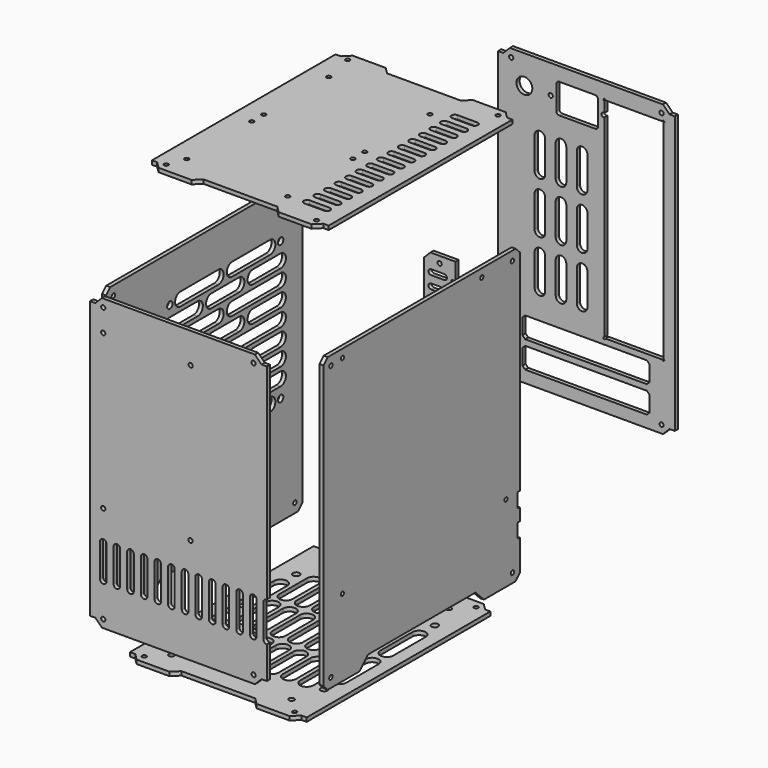
from build123d import *

# Parameters (mm, degrees)
F0_R      = 1.6
F1_DEPTH  = 3
F3_R      = 1.6
F4_DEPTH  = 3
F6_R      = 1.6
F7_DEPTH  = 3
F9_R      = 1.5
F9_W      = 2
F9_H      = 11
F10_DEPTH = 25
F12_R     = 1.6
F13_DEPTH = 3
F15_R     = 2.55
F16_DEPTH = 25
F18_R     = 1.6
F19_DEPTH = 3
F22_R     = 1.6
F23_DEPTH = 3
F26_R     = 1.6
F27_DEPTH = 3
F29_W     = 96.4
F29_H     = 15.9
F30_R     = 6
F30_R_2   = 1.6
F31_DEPTH = 25
F32_SIZE  = 2
F33_R     = 1.6
F34_DEPTH = 25
F35_R     = 2.55
F35_R_2   = 2
F36_DEPTH = 25
F37_R     = 1.6
F38_DEPTH = 3
F39_SIZE  = 0.5


# Not quite as in the source:
# - a feature names something its author has since deleted; it is built from what else it names


with BuildPart() as f1:
    # F0 (on Front) → F1 (new body)
    with BuildSketch(Plane.XZ):
        Polygon((-72.4445467208, 96.6760702261), (-76.4445467208, 96.6760702261), (-76.4445467208, -8.3239297739), (57.5554532792, -8.3239297739), (57.5554532792, 96.6760702261), (53.5554532792, 96.6760702261), (48.5554532792, 101.6760702261), (-67.4445467208, 101.6760702261), align=None)
        with Locations((-66.4445467208, 95.6760702261)):
            Circle(F0_R, mode=Mode.SUBTRACT)
        with Locations((47.5554532792, 95.6760702261)):
            Circle(F0_R, mode=Mode.SUBTRACT)
    extrude(amount=F1_DEPTH)

    # F2: F1 across face


with BuildPart() as f1_1:
    add(f1.part)
    add(f1.part.mirror(Plane(origin=(-9.4445467208, -1.5, -8.3239297739), x_dir=(1, 0, 0), z_dir=(0, 0, -1))))

    # F3 (on face) → F4 (cut)
    with BuildSketch(Plane.XZ.offset(3)):
        with Locations((-0.2445467208, 78.6760702261)):
            Circle(F3_R)
        with Locations((-66.4445467208, 78.6760702261)):
            Circle(F3_R)
        with Locations((-66.4445467208, -38.3239297739)):
            Circle(F3_R)
        with Locations((-0.2445467208, -38.3239297739)):
            Circle(F3_R)
        with BuildLine():
            ThreePointArc((-68.9445467208, -86.3239297739), (-66.4445467208, -88.8239297739), (-63.9445467208, -86.3239297739))
            Line((-63.9445467208, -86.3239297739), (-63.9445467208, -61.3239297739))
            ThreePointArc((-63.9445467208, -61.3239297739), (-66.4445467208, -58.8239297739), (-68.9445467208, -61.3239297739))
            Line((-68.9445467208, -61.3239297739), (-68.9445467208, -86.3239297739))
        make_face()
        with BuildLine():
            ThreePointArc((-58.6115467208, -86.3239297739), (-56.1115467208, -88.8239297739), (-53.6115467208, -86.3239297739))
            Line((-53.6115467208, -86.3239297739), (-53.6115467208, -61.3239297739))
            ThreePointArc((-53.6115467208, -61.3239297739), (-56.1115467208, -58.8239297739), (-58.6115467208, -61.3239297739))
            Line((-58.6115467208, -61.3239297739), (-58.6115467208, -86.3239297739))
        make_face()
        with BuildLine():
            ThreePointArc((-48.2785467208, -86.3239297739), (-45.7785467208, -88.8239297739), (-43.2785467208, -86.3239297739))
            Line((-43.2785467208, -86.3239297739), (-43.2785467208, -61.3239297739))
            ThreePointArc((-43.2785467208, -61.3239297739), (-45.7785467208, -58.8239297739), (-48.2785467208, -61.3239297739))
            Line((-48.2785467208, -61.3239297739), (-48.2785467208, -86.3239297739))
        make_face()
        with BuildLine():
            ThreePointArc((-37.9455467208, -86.3239297739), (-35.4455467208, -88.8239297739), (-32.9455467208, -86.3239297739))
            Line((-32.9455467208, -86.3239297739), (-32.9455467208, -61.3239297739))
            ThreePointArc((-32.9455467208, -61.3239297739), (-35.4455467208, -58.8239297739), (-37.9455467208, -61.3239297739))
            Line((-37.9455467208, -61.3239297739), (-37.9455467208, -86.3239297739))
        make_face()
        with BuildLine():
            ThreePointArc((-27.6125467208, -86.3239297739), (-25.1125467208, -88.8239297739), (-22.6125467208, -86.3239297739))
            Line((-22.6125467208, -86.3239297739), (-22.6125467208, -61.3239297739))
            ThreePointArc((-22.6125467208, -61.3239297739), (-25.1125467208, -58.8239297739), (-27.6125467208, -61.3239297739))
            Line((-27.6125467208, -61.3239297739), (-27.6125467208, -86.3239297739))
        make_face()
        with BuildLine():
            ThreePointArc((-17.2795467208, -86.3239297739), (-14.7795467208, -88.8239297739), (-12.2795467208, -86.3239297739))
            Line((-12.2795467208, -86.3239297739), (-12.2795467208, -61.3239297739))
            ThreePointArc((-12.2795467208, -61.3239297739), (-14.7795467208, -58.8239297739), (-17.2795467208, -61.3239297739))
            Line((-17.2795467208, -61.3239297739), (-17.2795467208, -86.3239297739))
        make_face()
        with BuildLine():
            ThreePointArc((-6.9465467208, -86.3239297739), (-4.4465467208, -88.8239297739), (-1.9465467208, -86.3239297739))
            Line((-1.9465467208, -86.3239297739), (-1.9465467208, -61.3239297739))
            ThreePointArc((-1.9465467208, -61.3239297739), (-4.4465467208, -58.8239297739), (-6.9465467208, -61.3239297739))
            Line((-6.9465467208, -61.3239297739), (-6.9465467208, -86.3239297739))
        make_face()
        with BuildLine():
            ThreePointArc((3.3864532792, -86.3239297739), (5.8864532792, -88.8239297739), (8.3864532792, -86.3239297739))
            Line((8.3864532792, -86.3239297739), (8.3864532792, -61.3239297739))
            ThreePointArc((8.3864532792, -61.3239297739), (5.8864532792, -58.8239297739), (3.3864532792, -61.3239297739))
            Line((3.3864532792, -61.3239297739), (3.3864532792, -86.3239297739))
        make_face()
        with BuildLine():
            ThreePointArc((13.7194532792, -86.3239297739), (16.2194532792, -88.8239297739), (18.7194532792, -86.3239297739))
            Line((18.7194532792, -86.3239297739), (18.7194532792, -61.3239297739))
            ThreePointArc((18.7194532792, -61.3239297739), (16.2194532792, -58.8239297739), (13.7194532792, -61.3239297739))
            Line((13.7194532792, -61.3239297739), (13.7194532792, -86.3239297739))
        make_face()
        with BuildLine():
            ThreePointArc((24.0524532792, -86.3239297739), (26.5524532792, -88.8239297739), (29.0524532792, -86.3239297739))
            Line((29.0524532792, -86.3239297739), (29.0524532792, -61.3239297739))
            ThreePointArc((29.0524532792, -61.3239297739), (26.5524532792, -58.8239297739), (24.0524532792, -61.3239297739))
            Line((24.0524532792, -61.3239297739), (24.0524532792, -86.3239297739))
        make_face()
        with BuildLine():
            ThreePointArc((34.3854532792, -86.3239297739), (36.8854532792, -88.8239297739), (39.3854532792, -86.3239297739))
            Line((39.3854532792, -86.3239297739), (39.3854532792, -61.3239297739))
            ThreePointArc((39.3854532792, -61.3239297739), (36.8854532792, -58.8239297739), (34.3854532792, -61.3239297739))
            Line((34.3854532792, -61.3239297739), (34.3854532792, -86.3239297739))
        make_face()
        with BuildLine():
            ThreePointArc((44.7184532792, -86.3239297739), (47.2184532792, -88.8239297739), (49.7184532792, -86.3239297739))
            Line((49.7184532792, -86.3239297739), (49.7184532792, -61.3239297739))
            ThreePointArc((49.7184532792, -61.3239297739), (47.2184532792, -58.8239297739), (44.7184532792, -61.3239297739))
            Line((44.7184532792, -61.3239297739), (44.7184532792, -86.3239297739))
        make_face()
        with BuildLine():
            ThreePointArc((55.0514532792, -86.3239297739), (57.5514532792, -88.8239297739), (60.0514532792, -86.3239297739))
            Line((60.0514532792, -86.3239297739), (60.0514532792, -61.3239297739))
            ThreePointArc((60.0514532792, -61.3239297739), (57.5514532792, -58.8239297739), (55.0514532792, -61.3239297739))
            Line((55.0514532792, -61.3239297739), (55.0514532792, -86.3239297739))
        make_face()
    extrude(amount=-F4_DEPTH, mode=Mode.SUBTRACT)


with BuildPart() as f7:
    # F6 (on offset) → F7 (new body)
    with BuildSketch(Plane.YZ.offset(80)):
        Polygon((200.9140200328, 100.6278687119), (22.9140200328, 100.6278687119), (18.9140200328, 96.6278687119), (18.9140200328, -10.3721312881), (204.9140200328, -10.3721312881), (204.9140200328, 96.6278687119), align=None)
        with Locations((25.9140200328, 93.6278687119)):
            Circle(F6_R, mode=Mode.SUBTRACT)
        with Locations((197.9140200328, 93.6278687119)):
            Circle(F6_R, mode=Mode.SUBTRACT)
    extrude(amount=F7_DEPTH)

    # F8: F7 across face


with BuildPart() as f7_1:
    add(f7.part)
    add(f7.part.mirror(Plane(origin=(81.5, 111.9140200328, -10.3721312881), x_dir=(1, 0, 0), z_dir=(0, 0, -1))))

    # F9 (on face) → F10 (cut)
    with BuildSketch(Plane(origin=(80, 0, 0), x_dir=(0, -1, 0), z_dir=(-1, 0, 0))):
        with Locations((-191.7140200328, -62.9721312881)):
            Circle(F9_R)
        with Locations((-36.8140200328, -62.9721312881)):
            Circle(F9_R)
        with Locations((-168.9140200328, 94.4278687119)):
            Circle(F9_R)
        with Locations((-36.8140200328, 94.4278687119)):
            Circle(F9_R)
        Polygon((-170.9140200328, -121.3721312881), (-52.9140200328, -121.3721312881), (-60.9140200328, -113.3721312881), (-162.9140200328, -113.3721312881), align=None)
        with Locations((-203.9140200328, -68.0721312881)):
            Rectangle(F9_W, F9_H)
        with Locations((-203.9140200328, -88.3721312881)):
            Rectangle(F9_W, F9_H)
    extrude(amount=-F10_DEPTH, mode=Mode.SUBTRACT)

    # F39
    f39_edges = [f7_1.edges().sort_by_distance(p)[0] for p in [
        (81.5, 202.91402, -93.872131),
        (81.5, 202.91402, -73.572131),
        (81.5, 202.91402, -62.572131),
        (81.5, 202.91402, -82.872131),
    ]]
    chamfer(f39_edges, length=F39_SIZE)


with BuildPart() as f13:
    # F12 (on offset) → F13 (new body)
    with BuildSketch(Plane.YZ.offset(-96)):
        Polygon((218.7864820957, 80.4807467597), (214.7864820957, 84.4807467597), (36.7864820957, 84.4807467597), (32.7864820957, 80.4807467597), (32.7864820957, -26.5192532403), (218.7864820957, -26.5192532403), align=None)
        with Locations((39.7864820957, 77.4807467597)):
            Circle(F12_R, mode=Mode.SUBTRACT)
        with Locations((211.7864820957, 77.4807467597)):
            Circle(F12_R, mode=Mode.SUBTRACT)
    extrude(amount=F13_DEPTH)

    # F14: F13 across face


with BuildPart() as f13_1:
    add(f13.part)
    add(f13.part.mirror(Plane(origin=(-94.5, 125.7864820957, -26.5192532403), x_dir=(1, 0, 0), z_dir=(0, 0, -1))))

    # F15 (on face) → F16 (cut)
    with BuildSketch(Plane(origin=(-96, 0, 0), x_dir=(0, -1, 0), z_dir=(-1, 0, 0))):
        with Locations((-198.2864820957, 49.4807467597)):
            Circle(F15_R)
        with Locations((-93.2864820957, 49.4807467597)):
            Circle(F15_R)
        with BuildLine():
            ThreePointArc((-188.2864820957, 54.4807467597), (-193.2864820957, 49.4807467597), (-188.2864820957, 44.4807467597))
            Line((-188.2864820957, 44.4807467597), (-152.2864820957, 44.4807467597))
            ThreePointArc((-152.2864820957, 44.4807467597), (-147.2864820957, 49.4807467597), (-152.2864820957, 54.4807467597))
            Line((-152.2864820957, 54.4807467597), (-188.2864820957, 54.4807467597))
        make_face()
        with BuildLine():
            ThreePointArc((-139.2864820957, 54.4807467597), (-144.2864820957, 49.4807467597), (-139.2864820957, 44.4807467597))
            Line((-139.2864820957, 44.4807467597), (-103.2864820957, 44.4807467597))
            ThreePointArc((-103.2864820957, 44.4807467597), (-98.2864820957, 49.4807467597), (-103.2864820957, 54.4807467597))
            Line((-103.2864820957, 54.4807467597), (-139.2864820957, 54.4807467597))
        make_face()
        with BuildLine():
            ThreePointArc((-198.2864820957, 41.3557467597), (-203.2864820957, 36.3557467597), (-198.2864820957, 31.3557467597))
            Line((-198.2864820957, 31.3557467597), (-171.9531487624, 31.3557467597))
            ThreePointArc((-171.9531487624, 31.3557467597), (-166.9531487624, 36.3557467597), (-171.9531487624, 41.3557467597))
            Line((-171.9531487624, 41.3557467597), (-198.2864820957, 41.3557467597))
        make_face()
        with BuildLine():
            ThreePointArc((-158.9531487624, 41.3557467597), (-163.9531487624, 36.3557467597), (-158.9531487624, 31.3557467597))
            Line((-158.9531487624, 31.3557467597), (-132.6198154291, 31.3557467597))
            ThreePointArc((-132.6198154291, 31.3557467597), (-127.6198154291, 36.3557467597), (-132.6198154291, 41.3557467597))
            Line((-132.6198154291, 41.3557467597), (-158.9531487624, 41.3557467597))
        make_face()
        with BuildLine():
            ThreePointArc((-119.6198154291, 41.3557467597), (-124.6198154291, 36.3557467597), (-119.6198154291, 31.3557467597))
            Line((-119.6198154291, 31.3557467597), (-93.2864820957, 31.3557467597))
            ThreePointArc((-93.2864820957, 31.3557467597), (-88.2864820957, 36.3557467597), (-93.2864820957, 41.3557467597))
            Line((-93.2864820957, 41.3557467597), (-119.6198154291, 41.3557467597))
        make_face()
        with BuildLine():
            ThreePointArc((-198.2864820957, 28.2307467597), (-203.2864820957, 23.2307467597), (-198.2864820957, 18.2307467597))
            Line((-198.2864820957, 18.2307467597), (-152.2864820957, 18.2307467597))
            ThreePointArc((-152.2864820957, 18.2307467597), (-147.2864820957, 23.2307467597), (-152.2864820957, 28.2307467597))
            Line((-152.2864820957, 28.2307467597), (-198.2864820957, 28.2307467597))
        make_face()
        with BuildLine():
            ThreePointArc((-139.2864820957, 28.2307467597), (-144.2864820957, 23.2307467597), (-139.2864820957, 18.2307467597))
            Line((-139.2864820957, 18.2307467597), (-93.2864820957, 18.2307467597))
            ThreePointArc((-93.2864820957, 18.2307467597), (-88.2864820957, 23.2307467597), (-93.2864820957, 28.2307467597))
            Line((-93.2864820957, 28.2307467597), (-139.2864820957, 28.2307467597))
        make_face()
        with BuildLine():
            ThreePointArc((-198.2864820957, 15.1057467597), (-203.2864820957, 10.1057467597), (-198.2864820957, 5.1057467597))
            Line((-198.2864820957, 5.1057467597), (-171.9531487624, 5.1057467597))
            ThreePointArc((-171.9531487624, 5.1057467597), (-166.9531487624, 10.1057467597), (-171.9531487624, 15.1057467597))
            Line((-171.9531487624, 15.1057467597), (-198.2864820957, 15.1057467597))
        make_face()
        with BuildLine():
            ThreePointArc((-158.9531487624, 15.1057467597), (-163.9531487624, 10.1057467597), (-158.9531487624, 5.1057467597))
            Line((-158.9531487624, 5.1057467597), (-132.6198154291, 5.1057467597))
            ThreePointArc((-132.6198154291, 5.1057467597), (-127.6198154291, 10.1057467597), (-132.6198154291, 15.1057467597))
            Line((-132.6198154291, 15.1057467597), (-158.9531487624, 15.1057467597))
        make_face()
        with BuildLine():
            ThreePointArc((-119.6198154291, 15.1057467597), (-124.6198154291, 10.1057467597), (-119.6198154291, 5.1057467597))
            Line((-119.6198154291, 5.1057467597), (-93.2864820957, 5.1057467597))
            ThreePointArc((-93.2864820957, 5.1057467597), (-88.2864820957, 10.1057467597), (-93.2864820957, 15.1057467597))
            Line((-93.2864820957, 15.1057467597), (-119.6198154291, 15.1057467597))
        make_face()
        with BuildLine():
            ThreePointArc((-198.2864820957, 1.9807467597), (-203.2864820957, -3.0192532403), (-198.2864820957, -8.0192532403))
            Line((-198.2864820957, -8.0192532403), (-152.2864820957, -8.0192532403))
            ThreePointArc((-152.2864820957, -8.0192532403), (-147.2864820957, -3.0192532403), (-152.2864820957, 1.9807467597))
            Line((-152.2864820957, 1.9807467597), (-198.2864820957, 1.9807467597))
        make_face()
        with BuildLine():
            ThreePointArc((-139.2864820957, 1.9807467597), (-144.2864820957, -3.0192532403), (-139.2864820957, -8.0192532403))
            Line((-139.2864820957, -8.0192532403), (-93.2864820957, -8.0192532403))
            ThreePointArc((-93.2864820957, -8.0192532403), (-88.2864820957, -3.0192532403), (-93.2864820957, 1.9807467597))
            Line((-93.2864820957, 1.9807467597), (-139.2864820957, 1.9807467597))
        make_face()
        with BuildLine():
            ThreePointArc((-198.2864820957, -11.1442532403), (-203.2864820957, -16.1442532403), (-198.2864820957, -21.1442532403))
            Line((-198.2864820957, -21.1442532403), (-171.9531487624, -21.1442532403))
            ThreePointArc((-171.9531487624, -21.1442532403), (-166.9531487624, -16.1442532403), (-171.9531487624, -11.1442532403))
            Line((-171.9531487624, -11.1442532403), (-198.2864820957, -11.1442532403))
        make_face()
        with BuildLine():
            ThreePointArc((-158.9531487624, -11.1442532403), (-163.9531487624, -16.1442532403), (-158.9531487624, -21.1442532403))
            Line((-158.9531487624, -21.1442532403), (-132.6198154291, -21.1442532403))
            ThreePointArc((-132.6198154291, -21.1442532403), (-127.6198154291, -16.1442532403), (-132.6198154291, -11.1442532403))
            Line((-132.6198154291, -11.1442532403), (-158.9531487624, -11.1442532403))
        make_face()
        with BuildLine():
            ThreePointArc((-119.6198154291, -11.1442532403), (-124.6198154291, -16.1442532403), (-119.6198154291, -21.1442532403))
            Line((-119.6198154291, -21.1442532403), (-93.2864820957, -21.1442532403))
            ThreePointArc((-93.2864820957, -21.1442532403), (-88.2864820957, -16.1442532403), (-93.2864820957, -11.1442532403))
            Line((-93.2864820957, -11.1442532403), (-119.6198154291, -11.1442532403))
        make_face()
        with BuildLine():
            ThreePointArc((-198.2864820957, -24.2692532403), (-203.2864820957, -29.2692532403), (-198.2864820957, -34.2692532403))
            Line((-198.2864820957, -34.2692532403), (-152.2864820957, -34.2692532403))
            ThreePointArc((-152.2864820957, -34.2692532403), (-147.2864820957, -29.2692532403), (-152.2864820957, -24.2692532403))
            Line((-152.2864820957, -24.2692532403), (-198.2864820957, -24.2692532403))
        make_face()
        with BuildLine():
            ThreePointArc((-139.2864820957, -24.2692532403), (-144.2864820957, -29.2692532403), (-139.2864820957, -34.2692532403))
            Line((-139.2864820957, -34.2692532403), (-93.2864820957, -34.2692532403))
            ThreePointArc((-93.2864820957, -34.2692532403), (-88.2864820957, -29.2692532403), (-93.2864820957, -24.2692532403))
            Line((-93.2864820957, -24.2692532403), (-139.2864820957, -24.2692532403))
        make_face()
        with BuildLine():
            ThreePointArc((-198.2864820957, -37.3942532403), (-203.2864820957, -42.3942532403), (-198.2864820957, -47.3942532403))
            Line((-198.2864820957, -47.3942532403), (-171.9531487624, -47.3942532403))
            ThreePointArc((-171.9531487624, -47.3942532403), (-166.9531487624, -42.3942532403), (-171.9531487624, -37.3942532403))
            Line((-171.9531487624, -37.3942532403), (-198.2864820957, -37.3942532403))
        make_face()
        with BuildLine():
            ThreePointArc((-158.9531487624, -37.3942532403), (-163.9531487624, -42.3942532403), (-158.9531487624, -47.3942532403))
            Line((-158.9531487624, -47.3942532403), (-132.6198154291, -47.3942532403))
            ThreePointArc((-132.6198154291, -47.3942532403), (-127.6198154291, -42.3942532403), (-132.6198154291, -37.3942532403))
            Line((-132.6198154291, -37.3942532403), (-158.9531487624, -37.3942532403))
        make_face()
        with BuildLine():
            ThreePointArc((-119.6198154291, -37.3942532403), (-124.6198154291, -42.3942532403), (-119.6198154291, -47.3942532403))
            Line((-119.6198154291, -47.3942532403), (-93.2864820957, -47.3942532403))
            ThreePointArc((-93.2864820957, -47.3942532403), (-88.2864820957, -42.3942532403), (-93.2864820957, -37.3942532403))
            Line((-93.2864820957, -37.3942532403), (-119.6198154291, -37.3942532403))
        make_face()
        with BuildLine():
            ThreePointArc((-188.2864820957, -50.5192532403), (-193.2864820957, -55.5192532403), (-188.2864820957, -60.5192532403))
            Line((-188.2864820957, -60.5192532403), (-152.2864820957, -60.5192532403))
            ThreePointArc((-152.2864820957, -60.5192532403), (-147.2864820957, -55.5192532403), (-152.2864820957, -50.5192532403))
            Line((-152.2864820957, -50.5192532403), (-188.2864820957, -50.5192532403))
        make_face()
        with BuildLine():
            ThreePointArc((-139.2864820957, -50.5192532403), (-144.2864820957, -55.5192532403), (-139.2864820957, -60.5192532403))
            Line((-139.2864820957, -60.5192532403), (-103.2864820957, -60.5192532403))
            ThreePointArc((-103.2864820957, -60.5192532403), (-98.2864820957, -55.5192532403), (-103.2864820957, -50.5192532403))
            Line((-103.2864820957, -50.5192532403), (-139.2864820957, -50.5192532403))
        make_face()
        with Locations((-198.2864820957, -55.5192532403)):
            Circle(F15_R)
        with Locations((-93.2864820957, -55.5192532403)):
            Circle(F15_R)
        Polygon((-166.7864820957, -129.5192532403), (-174.7864820957, -137.5192532403), (-76.7864820957, -137.5192532403), (-84.7864820957, -129.5192532403), align=None)
    extrude(amount=-F16_DEPTH, mode=Mode.SUBTRACT)


with BuildPart() as f19:
    # F18 (on offset) → F19 (new body)
    with BuildSketch(Plane.XY.offset(155)):
        Polygon((46.9777505851, 155.8661787467), (-87.0222494149, 155.8661787467), (-87.0222494149, 68.8661787467), (-83.0222494149, 68.8661787467), (-78.0222494149, 63.8661787467), (-53.0222494149, 63.8661787467), (-48.0222494149, 68.8661787467), (7.9777505851, 68.8661787467), (12.9777505851, 63.8661787467), (37.9777505851, 63.8661787467), (42.9777505851, 68.8661787467), (46.9777505851, 68.8661787467), align=None)
        with Locations((-77.0222494149, 69.8661787467)):
            Circle(F18_R, mode=Mode.SUBTRACT)
        with Locations((36.9777505851, 69.8661787467)):
            Circle(F18_R, mode=Mode.SUBTRACT)
    extrude(amount=F19_DEPTH)

    # F20: F19 across face


with BuildPart() as f19_1:
    add(f19.part)
    add(f19.part.mirror(Plane(origin=(-20.0222494149, 155.8661787467, 156.5), x_dir=(-1, 0, 0), z_dir=(0, 1, 0))))

    # F33 (on face) → F34 (cut)
    with BuildSketch(Plane.XY.offset(158)):
        with BuildLine():
            ThreePointArc((17.9777505851, 227.1161787467), (15.4777505851, 224.6161787467), (17.9777505851, 222.1161787467))
            Line((17.9777505851, 222.1161787467), (32.9777505851, 222.1161787467))
            ThreePointArc((32.9777505851, 222.1161787467), (35.4777505851, 224.6161787467), (32.9777505851, 227.1161787467))
            Line((32.9777505851, 227.1161787467), (17.9777505851, 227.1161787467))
        make_face()
        with BuildLine():
            ThreePointArc((17.9777505851, 217.1161787467), (15.4777505851, 214.6161787467), (17.9777505851, 212.1161787467))
            Line((17.9777505851, 212.1161787467), (32.9777505851, 212.1161787467))
            ThreePointArc((32.9777505851, 212.1161787467), (35.4777505851, 214.6161787467), (32.9777505851, 217.1161787467))
            Line((32.9777505851, 217.1161787467), (17.9777505851, 217.1161787467))
        make_face()
        with BuildLine():
            ThreePointArc((17.9777505851, 207.1161787467), (15.4777505851, 204.6161787467), (17.9777505851, 202.1161787467))
            Line((17.9777505851, 202.1161787467), (32.9777505851, 202.1161787467))
            ThreePointArc((32.9777505851, 202.1161787467), (35.4777505851, 204.6161787467), (32.9777505851, 207.1161787467))
            Line((32.9777505851, 207.1161787467), (17.9777505851, 207.1161787467))
        make_face()
        with BuildLine():
            ThreePointArc((17.9777505851, 197.1161787467), (15.4777505851, 194.6161787467), (17.9777505851, 192.1161787467))
            Line((17.9777505851, 192.1161787467), (32.9777505851, 192.1161787467))
            ThreePointArc((32.9777505851, 192.1161787467), (35.4777505851, 194.6161787467), (32.9777505851, 197.1161787467))
            Line((32.9777505851, 197.1161787467), (17.9777505851, 197.1161787467))
        make_face()
        with BuildLine():
            ThreePointArc((17.9777505851, 187.1161787467), (15.4777505851, 184.6161787467), (17.9777505851, 182.1161787467))
            Line((17.9777505851, 182.1161787467), (32.9777505851, 182.1161787467))
            ThreePointArc((32.9777505851, 182.1161787467), (35.4777505851, 184.6161787467), (32.9777505851, 187.1161787467))
            Line((32.9777505851, 187.1161787467), (17.9777505851, 187.1161787467))
        make_face()
        with BuildLine():
            ThreePointArc((17.9777505851, 177.1161787467), (15.4777505851, 174.6161787467), (17.9777505851, 172.1161787467))
            Line((17.9777505851, 172.1161787467), (32.9777505851, 172.1161787467))
            ThreePointArc((32.9777505851, 172.1161787467), (35.4777505851, 174.6161787467), (32.9777505851, 177.1161787467))
            Line((32.9777505851, 177.1161787467), (17.9777505851, 177.1161787467))
        make_face()
        with BuildLine():
            ThreePointArc((17.9777505851, 167.1161787467), (15.4777505851, 164.6161787467), (17.9777505851, 162.1161787467))
            Line((17.9777505851, 162.1161787467), (32.9777505851, 162.1161787467))
            ThreePointArc((32.9777505851, 162.1161787467), (35.4777505851, 164.6161787467), (32.9777505851, 167.1161787467))
            Line((32.9777505851, 167.1161787467), (17.9777505851, 167.1161787467))
        make_face()
        with BuildLine():
            ThreePointArc((17.9777505851, 157.1161787467), (15.4777505851, 154.6161787467), (17.9777505851, 152.1161787467))
            Line((17.9777505851, 152.1161787467), (32.9777505851, 152.1161787467))
            ThreePointArc((32.9777505851, 152.1161787467), (35.4777505851, 154.6161787467), (32.9777505851, 157.1161787467))
            Line((32.9777505851, 157.1161787467), (17.9777505851, 157.1161787467))
        make_face()
        with BuildLine():
            ThreePointArc((17.9777505851, 147.1161787467), (15.4777505851, 144.6161787467), (17.9777505851, 142.1161787467))
            Line((17.9777505851, 142.1161787467), (32.9777505851, 142.1161787467))
            ThreePointArc((32.9777505851, 142.1161787467), (35.4777505851, 144.6161787467), (32.9777505851, 147.1161787467))
            Line((32.9777505851, 147.1161787467), (17.9777505851, 147.1161787467))
        make_face()
        with BuildLine():
            ThreePointArc((17.9777505851, 137.1161787467), (15.4777505851, 134.6161787467), (17.9777505851, 132.1161787467))
            Line((17.9777505851, 132.1161787467), (32.9777505851, 132.1161787467))
            ThreePointArc((32.9777505851, 132.1161787467), (35.4777505851, 134.6161787467), (32.9777505851, 137.1161787467))
            Line((32.9777505851, 137.1161787467), (17.9777505851, 137.1161787467))
        make_face()
        with BuildLine():
            ThreePointArc((17.9777505851, 127.1161787467), (15.4777505851, 124.6161787467), (17.9777505851, 122.1161787467))
            Line((17.9777505851, 122.1161787467), (32.9777505851, 122.1161787467))
            ThreePointArc((32.9777505851, 122.1161787467), (35.4777505851, 124.6161787467), (32.9777505851, 127.1161787467))
            Line((32.9777505851, 127.1161787467), (17.9777505851, 127.1161787467))
        make_face()
        with BuildLine():
            ThreePointArc((17.9777505851, 117.1161787467), (15.4777505851, 114.6161787467), (17.9777505851, 112.1161787467))
            Line((17.9777505851, 112.1161787467), (32.9777505851, 112.1161787467))
            ThreePointArc((32.9777505851, 112.1161787467), (35.4777505851, 114.6161787467), (32.9777505851, 117.1161787467))
            Line((32.9777505851, 117.1161787467), (17.9777505851, 117.1161787467))
        make_face()
        with BuildLine():
            ThreePointArc((17.9777505851, 107.1161787467), (15.4777505851, 104.6161787467), (17.9777505851, 102.1161787467))
            Line((17.9777505851, 102.1161787467), (32.9777505851, 102.1161787467))
            ThreePointArc((32.9777505851, 102.1161787467), (35.4777505851, 104.6161787467), (32.9777505851, 107.1161787467))
            Line((32.9777505851, 107.1161787467), (17.9777505851, 107.1161787467))
        make_face()
        with BuildLine():
            ThreePointArc((17.9777505851, 97.1161787467), (15.4777505851, 94.6161787467), (17.9777505851, 92.1161787467))
            Line((17.9777505851, 92.1161787467), (32.9777505851, 92.1161787467))
            ThreePointArc((32.9777505851, 92.1161787467), (35.4777505851, 94.6161787467), (32.9777505851, 97.1161787467))
            Line((32.9777505851, 97.1161787467), (17.9777505851, 97.1161787467))
        make_face()
        with BuildLine():
            ThreePointArc((17.9777505851, 87.1161787467), (15.4777505851, 84.6161787467), (17.9777505851, 82.1161787467))
            Line((17.9777505851, 82.1161787467), (32.9777505851, 82.1161787467))
            ThreePointArc((32.9777505851, 82.1161787467), (35.4777505851, 84.6161787467), (32.9777505851, 87.1161787467))
            Line((32.9777505851, 87.1161787467), (17.9777505851, 87.1161787467))
        make_face()
        with Locations((4.5777505851, 83.0161787467)):
            Circle(F33_R)
        with Locations((4.5777505851, 144.7161787467)):
            Circle(F33_R)
        with Locations((-72.0222494149, 144.7161787467)):
            Circle(F33_R)
        with Locations((-72.0222494149, 83.0161787467)):
            Circle(F33_R)
        with Locations((-72.0222494149, 156.0161787467)):
            Circle(F33_R)
        with Locations((-72.0222494149, 217.7161787467)):
            Circle(F33_R)
        with Locations((4.5777505851, 217.7161787467)):
            Circle(F33_R)
        with Locations((4.5777505851, 156.0161787467)):
            Circle(F33_R)
    extrude(amount=-F34_DEPTH, mode=Mode.SUBTRACT)


with BuildPart() as f23:
    # F22 (on offset) → F23 (new body)
    with BuildSketch(Plane.XY.offset(-153)):
        Polygon((-68.9245462418, 30.4242391139), (-63.9245462418, 25.4242391139), (-38.9245462418, 25.4242391139), (-33.9245462418, 30.4242391139), (22.0754537582, 30.4242391139), (27.0754537582, 25.4242391139), (52.0754537582, 25.4242391139), (57.0754537582, 30.4242391139), (61.0754537582, 30.4242391139), (61.0754537582, 117.4242391139), (-72.9245462418, 117.4242391139), (-72.9245462418, 30.4242391139), align=None)
        with Locations((-62.9245462418, 31.4242391139)):
            Circle(F22_R, mode=Mode.SUBTRACT)
        with Locations((51.0754537582, 31.4242391139)):
            Circle(F22_R, mode=Mode.SUBTRACT)
    extrude(amount=F23_DEPTH)

    # F24: F23 across face


with BuildPart() as f23_1:
    add(f23.part)
    add(f23.part.mirror(Plane(origin=(-5.9245462418, 117.4242391139, -151.5), x_dir=(-1, 0, 0), z_dir=(0, 1, 0))))

    # F35 (on face) → F36 (cut)
    with BuildSketch(Plane(origin=(0, 0, -153), x_dir=(1, 0, 0), z_dir=(0, 0, -1))):
        with Locations((-58.4245462418, -169.9242391139)):
            Circle(F35_R)
        with Locations((-58.4245462418, -64.9242391139)):
            Circle(F35_R)
        with BuildLine():
            ThreePointArc((-63.4245462418, -154.9242391139), (-58.4245462418, -159.9242391139), (-53.4245462418, -154.9242391139))
            Line((-53.4245462418, -154.9242391139), (-53.4245462418, -121.4742391139))
            ThreePointArc((-53.4245462418, -121.4742391139), (-58.4245462418, -116.4742391139), (-63.4245462418, -121.4742391139))
            Line((-63.4245462418, -121.4742391139), (-63.4245462418, -154.9242391139))
        make_face()
        with BuildLine():
            ThreePointArc((-63.4245462418, -108.3742391139), (-58.4245462418, -113.3742391139), (-53.4245462418, -108.3742391139))
            Line((-53.4245462418, -108.3742391139), (-53.4245462418, -74.9242391139))
            ThreePointArc((-53.4245462418, -74.9242391139), (-58.4245462418, -69.9242391139), (-63.4245462418, -74.9242391139))
            Line((-63.4245462418, -74.9242391139), (-63.4245462418, -108.3742391139))
        make_face()
        with BuildLine():
            ThreePointArc((41.5754537582, -154.9242391139), (46.5754537582, -159.9242391139), (51.5754537582, -154.9242391139))
            Line((51.5754537582, -154.9242391139), (51.5754537582, -124.4242391139))
            ThreePointArc((51.5754537582, -124.4242391139), (46.5754537582, -119.4242391139), (41.5754537582, -124.4242391139))
            Line((41.5754537582, -124.4242391139), (41.5754537582, -154.9242391139))
        make_face()
        with BuildLine():
            ThreePointArc((41.5754537582, -110.4242391139), (46.5754537582, -115.4242391139), (51.5754537582, -110.4242391139))
            Line((51.5754537582, -110.4242391139), (51.5754537582, -79.9242391139))
            ThreePointArc((51.5754537582, -79.9242391139), (46.5754537582, -74.9242391139), (41.5754537582, -79.9242391139))
            Line((41.5754537582, -79.9242391139), (41.5754537582, -110.4242391139))
        make_face()
        with Locations((46.5754537582, -169.9242391139)):
            Circle(F35_R)
        with Locations((46.5754537582, -64.9242391139)):
            Circle(F35_R)
        with BuildLine():
            ThreePointArc((-50.2995462418, -169.9242391139), (-45.2995462418, -174.9242391139), (-40.2995462418, -169.9242391139))
            Line((-40.2995462418, -169.9242391139), (-40.2995462418, -143.6575724473))
            ThreePointArc((-40.2995462418, -143.6575724473), (-45.2995462418, -138.6575724473), (-50.2995462418, -143.6575724473))
            Line((-50.2995462418, -143.6575724473), (-50.2995462418, -169.9242391139))
        make_face()
        with BuildLine():
            ThreePointArc((-50.2995462418, -130.5575724473), (-45.2995462418, -135.5575724473), (-40.2995462418, -130.5575724473))
            Line((-40.2995462418, -130.5575724473), (-40.2995462418, -104.2909057806))
            ThreePointArc((-40.2995462418, -104.2909057806), (-45.2995462418, -99.2909057806), (-50.2995462418, -104.2909057806))
            Line((-50.2995462418, -104.2909057806), (-50.2995462418, -130.5575724473))
        make_face()
        with BuildLine():
            ThreePointArc((-40.2995462418, -64.9242391139), (-45.2995462418, -59.9242391139), (-50.2995462418, -64.9242391139))
            Line((-50.2995462418, -64.9242391139), (-50.2995462418, -91.1909057806))
            ThreePointArc((-50.2995462418, -91.1909057806), (-45.2995462418, -96.1909057806), (-40.2995462418, -91.1909057806))
            Line((-40.2995462418, -91.1909057806), (-40.2995462418, -64.9242391139))
        make_face()
        with BuildLine():
            ThreePointArc((-37.1745462418, -130.5575724473), (-32.1745462418, -135.5575724473), (-27.1745462418, -130.5575724473))
            Line((-27.1745462418, -130.5575724473), (-27.1745462418, -104.2909057806))
            ThreePointArc((-27.1745462418, -104.2909057806), (-32.1745462418, -99.2909057806), (-37.1745462418, -104.2909057806))
            Line((-37.1745462418, -104.2909057806), (-37.1745462418, -130.5575724473))
        make_face()
        with BuildLine():
            ThreePointArc((-27.1745462418, -143.6575724473), (-32.1745462418, -138.6575724473), (-37.1745462418, -143.6575724473))
            Line((-37.1745462418, -143.6575724473), (-37.1745462418, -169.9242391139))
            ThreePointArc((-37.1745462418, -169.9242391139), (-32.1745462418, -174.9242391139), (-27.1745462418, -169.9242391139))
            Line((-27.1745462418, -169.9242391139), (-27.1745462418, -143.6575724473))
        make_face()
        with BuildLine():
            ThreePointArc((-27.1745462418, -64.9242391139), (-32.1745462418, -59.9242391139), (-37.1745462418, -64.9242391139))
            Line((-37.1745462418, -64.9242391139), (-37.1745462418, -91.1909057806))
            ThreePointArc((-37.1745462418, -91.1909057806), (-32.1745462418, -96.1909057806), (-27.1745462418, -91.1909057806))
            Line((-27.1745462418, -91.1909057806), (-27.1745462418, -64.9242391139))
        make_face()
        with BuildLine():
            ThreePointArc((-24.0495462418, -130.5575724473), (-19.0495462418, -135.5575724473), (-14.0495462418, -130.5575724473))
            Line((-14.0495462418, -130.5575724473), (-14.0495462418, -104.2909057806))
            ThreePointArc((-14.0495462418, -104.2909057806), (-19.0495462418, -99.2909057806), (-24.0495462418, -104.2909057806))
            Line((-24.0495462418, -104.2909057806), (-24.0495462418, -130.5575724473))
        make_face()
        with BuildLine():
            ThreePointArc((-14.0495462418, -143.6575724473), (-19.0495462418, -138.6575724473), (-24.0495462418, -143.6575724473))
            Line((-24.0495462418, -143.6575724473), (-24.0495462418, -169.9242391139))
            ThreePointArc((-24.0495462418, -169.9242391139), (-19.0495462418, -174.9242391139), (-14.0495462418, -169.9242391139))
            Line((-14.0495462418, -169.9242391139), (-14.0495462418, -143.6575724473))
        make_face()
        with BuildLine():
            ThreePointArc((-14.0495462418, -64.9242391139), (-19.0495462418, -59.9242391139), (-24.0495462418, -64.9242391139))
            Line((-24.0495462418, -64.9242391139), (-24.0495462418, -91.1909057806))
            ThreePointArc((-24.0495462418, -91.1909057806), (-19.0495462418, -96.1909057806), (-14.0495462418, -91.1909057806))
            Line((-14.0495462418, -91.1909057806), (-14.0495462418, -64.9242391139))
        make_face()
        with BuildLine():
            ThreePointArc((-10.9245462418, -130.5575724473), (-5.9245462418, -135.5575724473), (-0.9245462418, -130.5575724473))
            Line((-0.9245462418, -130.5575724473), (-0.9245462418, -104.2909057806))
            ThreePointArc((-0.9245462418, -104.2909057806), (-5.9245462418, -99.2909057806), (-10.9245462418, -104.2909057806))
            Line((-10.9245462418, -104.2909057806), (-10.9245462418, -130.5575724473))
        make_face()
        with BuildLine():
            ThreePointArc((-0.9245462418, -143.6575724473), (-5.9245462418, -138.6575724473), (-10.9245462418, -143.6575724473))
            Line((-10.9245462418, -143.6575724473), (-10.9245462418, -169.9242391139))
            ThreePointArc((-10.9245462418, -169.9242391139), (-5.9245462418, -174.9242391139), (-0.9245462418, -169.9242391139))
            Line((-0.9245462418, -169.9242391139), (-0.9245462418, -143.6575724473))
        make_face()
        with BuildLine():
            ThreePointArc((-0.9245462418, -64.9242391139), (-5.9245462418, -59.9242391139), (-10.9245462418, -64.9242391139))
            Line((-10.9245462418, -64.9242391139), (-10.9245462418, -91.1909057806))
            ThreePointArc((-10.9245462418, -91.1909057806), (-5.9245462418, -96.1909057806), (-0.9245462418, -91.1909057806))
            Line((-0.9245462418, -91.1909057806), (-0.9245462418, -64.9242391139))
        make_face()
        with BuildLine():
            ThreePointArc((2.2004537582, -130.5575724473), (7.2004537582, -135.5575724473), (12.2004537582, -130.5575724473))
            Line((12.2004537582, -130.5575724473), (12.2004537582, -104.2909057806))
            ThreePointArc((12.2004537582, -104.2909057806), (7.2004537582, -99.2909057806), (2.2004537582, -104.2909057806))
            Line((2.2004537582, -104.2909057806), (2.2004537582, -130.5575724473))
        make_face()
        with BuildLine():
            ThreePointArc((12.2004537582, -143.6575724473), (7.2004537582, -138.6575724473), (2.2004537582, -143.6575724473))
            Line((2.2004537582, -143.6575724473), (2.2004537582, -169.9242391139))
            ThreePointArc((2.2004537582, -169.9242391139), (7.2004537582, -174.9242391139), (12.2004537582, -169.9242391139))
            Line((12.2004537582, -169.9242391139), (12.2004537582, -143.6575724473))
        make_face()
        with BuildLine():
            ThreePointArc((12.2004537582, -64.9242391139), (7.2004537582, -59.9242391139), (2.2004537582, -64.9242391139))
            Line((2.2004537582, -64.9242391139), (2.2004537582, -91.1909057806))
            ThreePointArc((2.2004537582, -91.1909057806), (7.2004537582, -96.1909057806), (12.2004537582, -91.1909057806))
            Line((12.2004537582, -91.1909057806), (12.2004537582, -64.9242391139))
        make_face()
        with BuildLine():
            ThreePointArc((15.3254537582, -130.5575724473), (20.3254537582, -135.5575724473), (25.3254537582, -130.5575724473))
            Line((25.3254537582, -130.5575724473), (25.3254537582, -104.2909057806))
            ThreePointArc((25.3254537582, -104.2909057806), (20.3254537582, -99.2909057806), (15.3254537582, -104.2909057806))
            Line((15.3254537582, -104.2909057806), (15.3254537582, -130.5575724473))
        make_face()
        with BuildLine():
            ThreePointArc((25.3254537582, -143.6575724473), (20.3254537582, -138.6575724473), (15.3254537582, -143.6575724473))
            Line((15.3254537582, -143.6575724473), (15.3254537582, -169.9242391139))
            ThreePointArc((15.3254537582, -169.9242391139), (20.3254537582, -174.9242391139), (25.3254537582, -169.9242391139))
            Line((25.3254537582, -169.9242391139), (25.3254537582, -143.6575724473))
        make_face()
        with BuildLine():
            ThreePointArc((25.3254537582, -64.9242391139), (20.3254537582, -59.9242391139), (15.3254537582, -64.9242391139))
            Line((15.3254537582, -64.9242391139), (15.3254537582, -91.1909057806))
            ThreePointArc((15.3254537582, -91.1909057806), (20.3254537582, -96.1909057806), (25.3254537582, -91.1909057806))
            Line((25.3254537582, -91.1909057806), (25.3254537582, -64.9242391139))
        make_face()
        with BuildLine():
            ThreePointArc((28.4504537582, -130.5575724473), (33.4504537582, -135.5575724473), (38.4504537582, -130.5575724473))
            Line((38.4504537582, -130.5575724473), (38.4504537582, -104.2909057806))
            ThreePointArc((38.4504537582, -104.2909057806), (33.4504537582, -99.2909057806), (28.4504537582, -104.2909057806))
            Line((28.4504537582, -104.2909057806), (28.4504537582, -130.5575724473))
        make_face()
        with BuildLine():
            ThreePointArc((38.4504537582, -143.6575724473), (33.4504537582, -138.6575724473), (28.4504537582, -143.6575724473))
            Line((28.4504537582, -143.6575724473), (28.4504537582, -169.9242391139))
            ThreePointArc((28.4504537582, -169.9242391139), (33.4504537582, -174.9242391139), (38.4504537582, -169.9242391139))
            Line((38.4504537582, -169.9242391139), (38.4504537582, -143.6575724473))
        make_face()
        with BuildLine():
            ThreePointArc((38.4504537582, -64.9242391139), (33.4504537582, -59.9242391139), (28.4504537582, -64.9242391139))
            Line((28.4504537582, -64.9242391139), (28.4504537582, -91.1909057806))
            ThreePointArc((28.4504537582, -91.1909057806), (33.4504537582, -96.1909057806), (38.4504537582, -91.1909057806))
            Line((38.4504537582, -91.1909057806), (38.4504537582, -64.9242391139))
        make_face()
        with Locations((39.5754537582, -42.9242391139)):
            Circle(F35_R_2)
        with Locations((39.5754537582, -191.9242391139)):
            Circle(F35_R_2)
        with Locations((-51.4245462418, -42.9242391139)):
            Circle(F35_R_2)
        with Locations((-51.4245462418, -191.9242391139)):
            Circle(F35_R_2)
    extrude(amount=-F36_DEPTH, mode=Mode.SUBTRACT)


with BuildPart() as f27:
    # F26 (on offset) → F27 (new body)
    with BuildSketch(Plane.XZ.offset(-376)):
        Polygon((-64, 113.4973174244), (-68, 113.4973174244), (-68, 8.4973174244), (66, 8.4973174244), (66, 113.4973174244), (62, 113.4973174244), (57, 118.4973174244), (-59, 118.4973174244), align=None)
        with Locations((-58, 112.4973174244)):
            Circle(F26_R, mode=Mode.SUBTRACT)
        with Locations((56, 112.4973174244)):
            Circle(F26_R, mode=Mode.SUBTRACT)
    extrude(amount=F27_DEPTH)

    # F28: F27 across face


with BuildPart() as f27_1:
    add(f27.part)
    add(f27.part.mirror(Plane(origin=(-1, 374.5, 8.4973174244), x_dir=(1, 0, 0), z_dir=(0, 0, -1))))

    # F29 (on face) + F30 (on face) → F31 (cut)
    with BuildSketch(Plane(origin=(0, 376, 0), x_dir=(-1, 0, 0), z_dir=(0, 1, 0))):
        with Locations((1.3, -64.2026825756)):
            Rectangle(F29_W, F29_H)
        with Locations((1.3, -84.5026825756)):
            Rectangle(F29_W, F29_H)
        Polygon((-12.6, 106.3473174244), (-12.6, 107.0973174244), (-13.35, 107.0973174244), (-56.55, 107.0973174244), (-57.3, 107.0973174244), (-57.3, 106.3473174244), (-57.3, -51.1526825756), (-57.3, -51.9026825756), (-56.55, -51.9026825756), (-13.35, -51.9026825756), (-12.6, -51.9026825756), (-12.6, -51.1526825756), align=None)
        with BuildLine():
            Line((-13.35, 107.0973174244), (-12.6, 107.0973174244))
            Line((-12.6, 107.0973174244), (-12.6, 106.3473174244))
            ThreePointArc((-12.6, 106.3473174244), (-12.0696699141, 107.6276475103), (-13.35, 107.0973174244))
        make_face()
        with BuildLine():
            Line((-57.3, 107.0973174244), (-56.55, 107.0973174244))
            ThreePointArc((-56.55, 107.0973174244), (-57.8303300859, 107.6276475103), (-57.3, 106.3473174244))
            Line((-57.3, 106.3473174244), (-57.3, 107.0973174244))
        make_face()
        with BuildLine():
            ThreePointArc((-13.35, -51.9026825756), (-12.0696699141, -52.4330126615), (-12.6, -51.1526825756))
            Line((-12.6, -51.1526825756), (-12.6, -51.9026825756))
            Line((-12.6, -51.9026825756), (-13.35, -51.9026825756))
        make_face()
        with BuildLine():
            Line((-57.3, -51.9026825756), (-57.3, -51.1526825756))
            ThreePointArc((-57.3, -51.1526825756), (-57.8303300859, -52.4330126615), (-56.55, -51.9026825756))
            Line((-56.55, -51.9026825756), (-57.3, -51.9026825756))
        make_face()
        Polygon((60.5, -51.7526825756), (54.5, -51.7526825756), (54.5, -91.7526825756), (72.5, -91.7526825756), (72.5, -51.7526825756), (72.5, -48.7526825756), (63.5, -48.7526825756), align=None)
    with BuildSketch(Plane(origin=(0, 376, 0), x_dir=(-1, 0, 0), z_dir=(0, 1, 0))):
        with BuildLine():
            ThreePointArc((8.25, 66.4973174244), (4.25, 70.4973174244), (0.25, 66.4973174244))
            Line((0.25, 66.4973174244), (0.25, 42.4973174244))
            ThreePointArc((0.25, 42.4973174244), (4.25, 38.4973174244), (8.25, 42.4973174244))
            Line((8.25, 42.4973174244), (8.25, 66.4973174244))
        make_face()
        with BuildLine():
            ThreePointArc((8.25, 27.4973174244), (4.25, 31.4973174244), (0.25, 27.4973174244))
            Line((0.25, 27.4973174244), (0.25, 3.4973174244))
            ThreePointArc((0.25, 3.4973174244), (4.25, -0.5026825756), (8.25, 3.4973174244))
            Line((8.25, 3.4973174244), (8.25, 27.4973174244))
        make_face()
        with BuildLine():
            ThreePointArc((8.25, -11.5026825756), (4.25, -7.5026825756), (0.25, -11.5026825756))
            Line((0.25, -11.5026825756), (0.25, -35.5026825756))
            ThreePointArc((0.25, -35.5026825756), (4.25, -39.5026825756), (8.25, -35.5026825756))
            Line((8.25, -35.5026825756), (8.25, -11.5026825756))
        make_face()
        with BuildLine():
            ThreePointArc((24.25, 27.4973174244), (20.25, 31.4973174244), (16.25, 27.4973174244))
            Line((16.25, 27.4973174244), (16.25, 3.4973174244))
            ThreePointArc((16.25, 3.4973174244), (20.25, -0.5026825756), (24.25, 3.4973174244))
            Line((24.25, 3.4973174244), (24.25, 27.4973174244))
        make_face()
        with BuildLine():
            ThreePointArc((24.25, -11.5026825756), (20.25, -7.5026825756), (16.25, -11.5026825756))
            Line((16.25, -11.5026825756), (16.25, -35.5026825756))
            ThreePointArc((16.25, -35.5026825756), (20.25, -39.5026825756), (24.25, -35.5026825756))
            Line((24.25, -35.5026825756), (24.25, -11.5026825756))
        make_face()
        with BuildLine():
            ThreePointArc((24.25, 66.4973174244), (20.25, 70.4973174244), (16.25, 66.4973174244))
            Line((16.25, 66.4973174244), (16.25, 42.4973174244))
            ThreePointArc((16.25, 42.4973174244), (20.25, 38.4973174244), (24.25, 42.4973174244))
            Line((24.25, 42.4973174244), (24.25, 66.4973174244))
        make_face()
        with BuildLine():
            ThreePointArc((40.25, 27.4973174244), (36.25, 31.4973174244), (32.25, 27.4973174244))
            Line((32.25, 27.4973174244), (32.25, 3.4973174244))
            ThreePointArc((32.25, 3.4973174244), (36.25, -0.5026825756), (40.25, 3.4973174244))
            Line((40.25, 3.4973174244), (40.25, 27.4973174244))
        make_face()
        with BuildLine():
            ThreePointArc((40.25, -11.5026825756), (36.25, -7.5026825756), (32.25, -11.5026825756))
            Line((32.25, -11.5026825756), (32.25, -35.5026825756))
            ThreePointArc((32.25, -35.5026825756), (36.25, -39.5026825756), (40.25, -35.5026825756))
            Line((40.25, -35.5026825756), (40.25, -11.5026825756))
        make_face()
        with BuildLine():
            ThreePointArc((40.25, 66.4973174244), (36.25, 70.4973174244), (32.25, 66.4973174244))
            Line((32.25, 66.4973174244), (32.25, 42.4973174244))
            ThreePointArc((32.25, 42.4973174244), (36.25, 38.4973174244), (40.25, 42.4973174244))
            Line((40.25, 42.4973174244), (40.25, 66.4973174244))
        make_face()
        with Locations((48, 96.8473174244)):
            Circle(F30_R)
        with BuildLine():
            Line((21.75, 108.0973174244), (-5.75, 108.0973174244))
            ThreePointArc((-5.75, 108.0973174244), (-7.1642135624, 107.5115309868), (-7.75, 106.0973174244))
            Line((-7.75, 106.0973174244), (-7.75, 87.5973174244))
            ThreePointArc((-7.75, 87.5973174244), (-7.1642135624, 86.183103862), (-5.75, 85.5973174244))
            Line((-5.75, 85.5973174244), (21.75, 85.5973174244))
            ThreePointArc((21.75, 85.5973174244), (23.1642135624, 86.183103862), (23.75, 87.5973174244))
            Line((23.75, 87.5973174244), (23.75, 106.0973174244))
            ThreePointArc((23.75, 106.0973174244), (23.1642135624, 107.5115309868), (21.75, 108.0973174244))
        make_face()
        with Locations((-12, 96.8473174244)):
            Circle(F30_R_2)
        with Locations((28, 96.8473174244)):
            Circle(F30_R_2)
    extrude(amount=-F31_DEPTH, mode=Mode.SUBTRACT)

    # F32
    f32_edges = [f27_1.edges().sort_by_distance(p)[0] for p in [
        (46.9, 374.5, -56.252683),
        (46.9, 374.5, -72.152683),
        (46.9, 374.5, -76.552683),
        (46.9, 374.5, -92.452683),
        (-49.5, 374.5, -92.452683),
        (-49.5, 374.5, -76.552683),
        (-49.5, 374.5, -72.152683),
        (-49.5, 374.5, -56.252683),
    ]]
    chamfer(f32_edges, length=F32_SIZE)


with BuildPart() as f38:
    # F37 (on offset) → F38 (new body)
    with BuildSketch(Plane.XZ.offset(-376)):
        Polygon((-100.2305700779, -49.5852892995), (-100.2305700779, -37.5852892995), (-119.2305700779, -37.5852892995), (-124.2305700779, -42.5852892995), (-124.2305700779, -95.5852892995), (-119.2305700779, -100.5852892995), (-100.2305700779, -100.5852892995), (-100.2305700779, -91.5852892995), (-101.2305700779, -90.5852892995), (-103.3305700779, -90.5852892995), (-103.3305700779, -50.5852892995), (-101.2305700779, -50.5852892995), align=None)
        with BuildLine():
            ThreePointArc((-118.7305700779, -90.5852892995), (-120.7305700779, -88.5852892995), (-118.7305700779, -86.5852892995))
            Line((-118.7305700779, -86.5852892995), (-108.7305700779, -86.5852892995))
            ThreePointArc((-108.7305700779, -86.5852892995), (-106.7305700779, -88.5852892995), (-108.7305700779, -90.5852892995))
            Line((-108.7305700779, -90.5852892995), (-118.7305700779, -90.5852892995))
        make_face(mode=Mode.SUBTRACT)
        with BuildLine():
            ThreePointArc((-118.7305700779, -81.0852892995), (-120.7305700779, -79.0852892995), (-118.7305700779, -77.0852892995))
            Line((-118.7305700779, -77.0852892995), (-108.7305700779, -77.0852892995))
            ThreePointArc((-108.7305700779, -77.0852892995), (-106.7305700779, -79.0852892995), (-108.7305700779, -81.0852892995))
            Line((-108.7305700779, -81.0852892995), (-118.7305700779, -81.0852892995))
        make_face(mode=Mode.SUBTRACT)
        with BuildLine():
            ThreePointArc((-118.7305700779, -71.5852892995), (-120.7305700779, -69.5852892995), (-118.7305700779, -67.5852892995))
            Line((-118.7305700779, -67.5852892995), (-108.7305700779, -67.5852892995))
            ThreePointArc((-108.7305700779, -67.5852892995), (-106.7305700779, -69.5852892995), (-108.7305700779, -71.5852892995))
            Line((-108.7305700779, -71.5852892995), (-118.7305700779, -71.5852892995))
        make_face(mode=Mode.SUBTRACT)
        with Locations((-112.2305700779, -95.5852892995)):
            Circle(F37_R, mode=Mode.SUBTRACT)
        with BuildLine():
            ThreePointArc((-118.7305700779, -62.0852892995), (-120.7305700779, -60.0852892995), (-118.7305700779, -58.0852892995))
            Line((-118.7305700779, -58.0852892995), (-108.7305700779, -58.0852892995))
            ThreePointArc((-108.7305700779, -58.0852892995), (-106.7305700779, -60.0852892995), (-108.7305700779, -62.0852892995))
            Line((-108.7305700779, -62.0852892995), (-118.7305700779, -62.0852892995))
        make_face(mode=Mode.SUBTRACT)
        with BuildLine():
            Line((-108.7305700779, -52.5852892995), (-118.7305700779, -52.5852892995))
            ThreePointArc((-118.7305700779, -52.5852892995), (-120.7305700779, -50.5852892995), (-118.7305700779, -48.5852892995))
            Line((-118.7305700779, -48.5852892995), (-108.7305700779, -48.5852892995))
            ThreePointArc((-108.7305700779, -48.5852892995), (-106.7305700779, -50.5852892995), (-108.7305700779, -52.5852892995))
        make_face(mode=Mode.SUBTRACT)
        with Locations((-112.2305700779, -42.5852892995)):
            Circle(F37_R, mode=Mode.SUBTRACT)
    extrude(amount=F38_DEPTH)


solid = Compound([f1_1.part, f7_1.part, f13_1.part, f19_1.part, f23_1.part, f27_1.part, f38.part])
